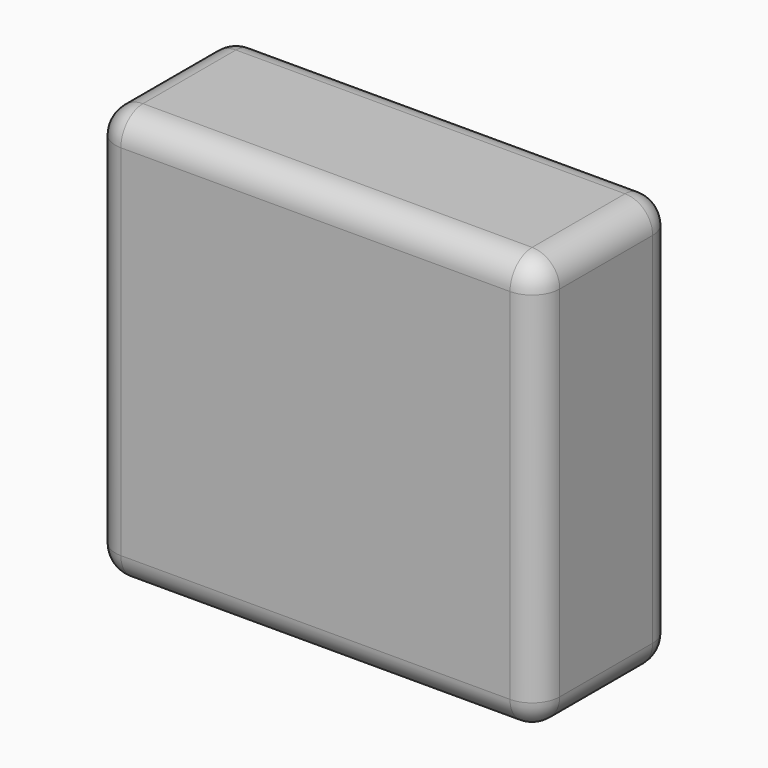
from build123d import *

# Parameters (mm, degrees)
F0_W     = 81.7405879498
F0_H     = 31.518612057
F1_DEPTH = 38.1
F2_R     = 5.08
F3_T     = -2.54


# Not quite as in the source:
# - a shell that OpenCascade refuses in one call is made with other operations: the cavity is built on its own and cut out


with BuildPart() as f1:
    # F0 (on Top) → F1 (new body, symmetric)
    with BuildSketch(Plane.XY):
        Rectangle(F0_W, F0_H)
    extrude(amount=F1_DEPTH, both=True)

    # F2
    f2_edges = [f1.edges().sort_by_distance(p)[0] for p in [
        (40.870294, -15.759306, 0),
        (0, -15.759306, 38.1),
        (-40.870294, -15.759306, 0),
        (0, -15.759306, -38.1),
        (-40.870294, 15.759306, 0),
        (-40.870294, 0, -38.1),
        (40.870294, 0, -38.1),
        (0, 15.759306, -38.1),
        (40.870294, 0, 38.1),
        (40.870294, 15.759306, 0),
        (0, 15.759306, 38.1),
        (-40.870294, 0, 38.1),
    ]]
    fillet(f2_edges, radius=F2_R)

    # F3: a shell. OpenCascade refuses it in one call, so the cavity is built on its own and cut out:
    # the body offset inwards by the wall thickness, plus a prism from it out through each open face.
    f3_core = offset(f1.part, amount=F3_T, mode=Mode.PRIVATE)
    f3_exits = [f3_core.faces().sort_by_distance(p)[0] for p in [
        (0, 13.219306, 0),
    ]]
    add(f3_core, mode=Mode.SUBTRACT)
    extrude(f3_exits, amount=-F3_T, mode=Mode.SUBTRACT)


solid = f1.part
